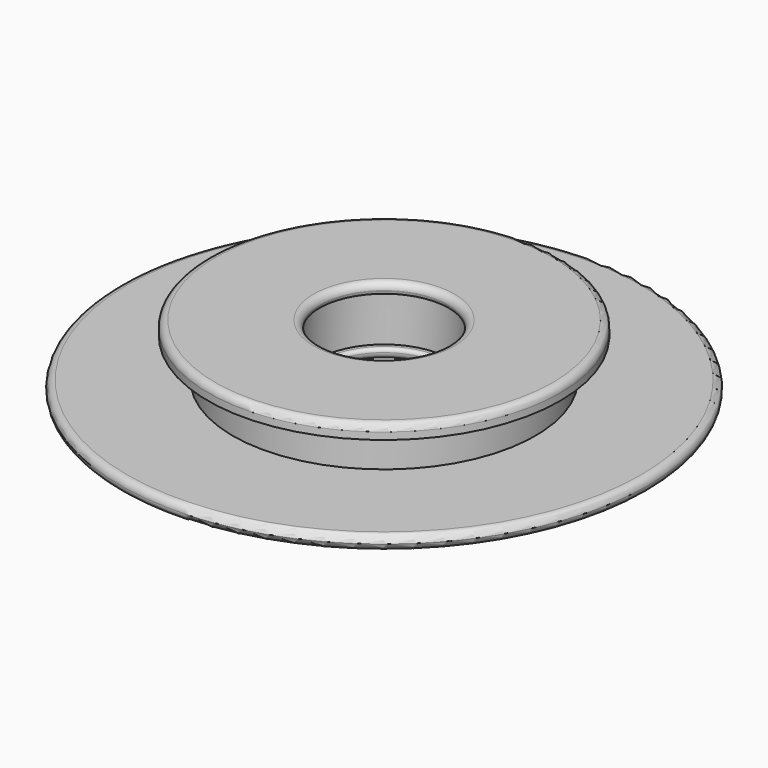
from build123d import *

# Parameters (mm, degrees)
F0_R     = 25
F0_R_2   = 9.5
F1_DEPTH = 9.5
F2_W     = 3.5
F2_H     = 5.5
F4_R     = 9.5
F4_R_2   = 8.5
F5_DEPTH = 1.5
F6_R     = 9.5
F6_R_2   = 9
F7_DEPTH = 1.6
F0_R_3   = 37.5
F8_DEPTH = 2
F9_R     = 0.99999
F10_R    = 0.49999


# Not quite as in the source:
# - a fillet or chamfer is up to 0.001 mm smaller than in the source, because OpenCascade refuses the exact size


with BuildPart() as f1:
    # F0 (on Top) → F1 (new body)
    with BuildSketch(Plane.XY):
        Circle(F0_R)
        Circle(F0_R_2, mode=Mode.SUBTRACT)
    extrude(amount=F1_DEPTH)

    # F2 (on Right) → F3 (revolve, cut)
    with BuildSketch(Plane.YZ):
        with Locations((23.25, 4.75)):
            Rectangle(F2_W, F2_H)
    revolve(axis=Axis((0, 0, 13.2580241188), (0, 0, 1)), mode=Mode.SUBTRACT)

    # F4 (on face) → F5 (join)
    with BuildSketch(Plane(origin=(0, 0, 0), x_dir=(1, 0, 0), z_dir=(0, 0, -1))):
        Circle(F4_R)
        Circle(F4_R_2, mode=Mode.SUBTRACT)
    extrude(amount=-F5_DEPTH)

    # F6 (on face) → F7 (join)
    with BuildSketch(Plane.XY.offset(9.5)):
        Circle(F6_R)
        Circle(F6_R_2, mode=Mode.SUBTRACT)
    extrude(amount=-F7_DEPTH)

    # F0 (on Top) → F8 (join)
    with BuildSketch(Plane.XY):
        Circle(F0_R_3)
        Circle(F0_R, mode=Mode.SUBTRACT)
    extrude(amount=F8_DEPTH)

    # F9 (radius 1 in the source; OpenCascade refuses exactly that, so slightly less here)
    f9_edges = [f1.edges().sort_by_distance(p)[0] for p in [
        (37.5, 0, 1),
        (-37.5, 0, 0),
        (-37.5, 0, 2),
        (-25, 0, 9.5),
        (-9, 0, 9.5),
        (-8.5, 0, 0),
    ]]
    fillet(f9_edges, radius=F9_R)

    # F10 (radius 0.5 in the source; OpenCascade refuses exactly that, so slightly less here)
    f10_edges = [f1.edges().sort_by_distance(p)[0] for p in [
        (-8.5, 0, 1.5),
        (-9, 0, 7.9),
    ]]
    fillet(f10_edges, radius=F10_R)


solid = f1.part
